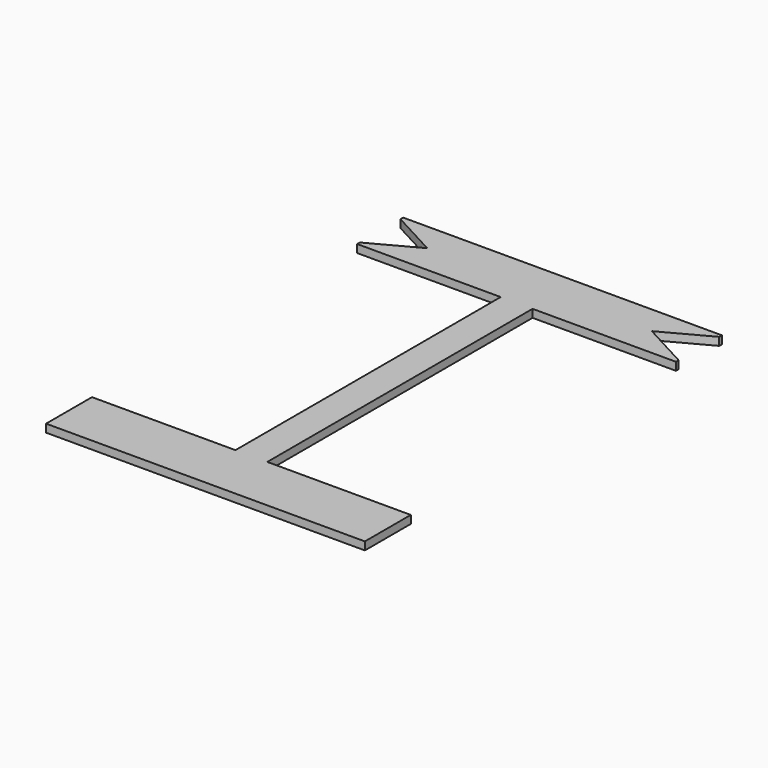
from build123d import *

# Parameters (mm, degrees)
F0_W     = 12.7
F0_H     = 132.08
F1_DEPTH = 3.175
F3_DEPTH = 25.4
F4_DEPTH = 25.4


# Not quite as in the source:
# - a feature names something its author has since deleted; it is built from what else it names


with BuildPart() as f1:
    # F0 (on Top) → F1 (new body)
    with BuildSketch(Plane.XY):
        Polygon((28.5549264625, 56.9072367892), (-98.4450735375, 56.9072367892), (-98.4450735375, 34.0472367892), (-41.2950735375, 34.0472367892), (-28.5950735375, 34.0472367892), (28.5549264625, 34.0472367892), align=None)
        with Locations((-34.9450735375, -31.9927632108)):
            Rectangle(F0_W, F0_H)
        Polygon((-41.2950735375, -98.0327632108), (-98.4450735375, -98.0327632108), (-98.4450735375, -120.8927632108), (28.5549264625, -120.8927632108), (28.5549264625, -98.0327632108), (-28.5950735375, -98.0327632108), align=None)
    extrude(amount=F1_DEPTH)

    # F2 (on face) → F3 (cut)
    with BuildSketch(Plane.XY.offset(3.175)):
        Polygon((28.5549264625, 45.4772367892), (9.7966708748, 45.4772367892), (28.5549264625, 35.3785827756), align=None)
        Polygon((-98.4450735375, 35.3785827756), (-79.6868179499, 45.4772367892), (-98.4450735375, 45.4772367892), align=None)
    extrude(amount=-F3_DEPTH, mode=Mode.SUBTRACT)

    # F2 (on face) → F4 (cut)
    with BuildSketch(Plane.XY.offset(3.175)):
        Polygon((28.5549264625, 55.5758908027), (9.7966708748, 45.4772367892), (28.5549264625, 45.4772367892), align=None)
        Polygon((-98.4450735375, 45.4772367892), (-79.6868179499, 45.4772367892), (-98.4450735375, 55.5758908027), align=None)
    extrude(amount=-F4_DEPTH, mode=Mode.SUBTRACT)


solid = f1.part
